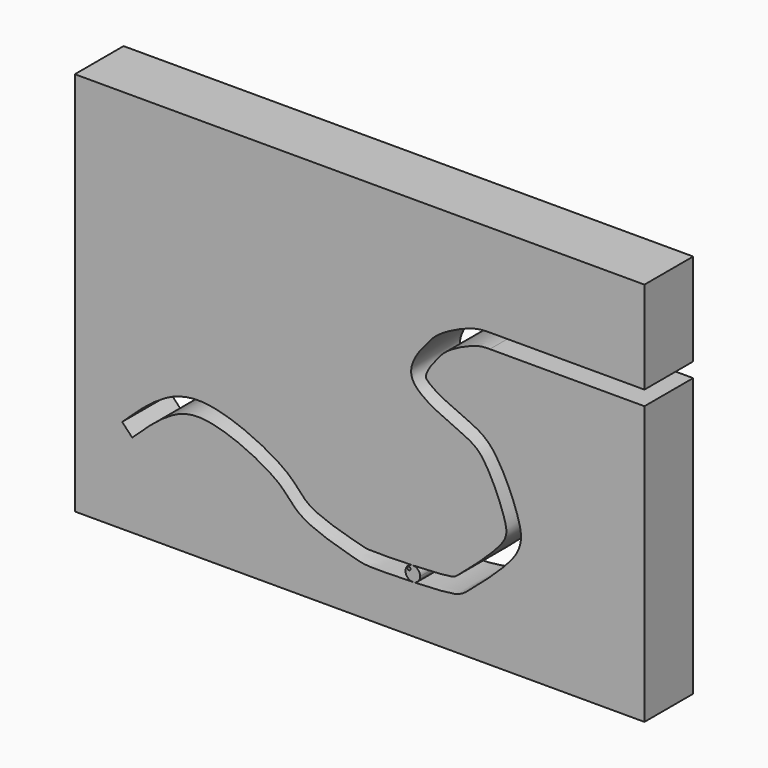
from build123d import *

# Parameters (mm, degrees)
F0_R     = 0.6651863413
F1_DEPTH = 25
F2_DEPTH = 25


# Not quite as in the source:
# - the dataset's text gives a spline's control points without its knots; the knots are read off the source's solid


with BuildPart() as f1:
    # F0 (on Front) → F1 (new body)
    with BuildSketch(Plane.XZ):
        with BuildLine():
            ThreePointArc((122.3084832169, -16.0360134831), (121.3921244993, -13.8776717571), (119.2028572127, -13.0378735352))
            ThreePointArc((119.2028572127, -13.0378735352), (116.3103432648, -16.1416393675), (119.4141089815, -19.0341534395))
            ThreePointArc((119.4141089815, -19.0341534395), (121.4668248597, -18.1196548518), (122.3084832169, -16.0360134831))
        make_face()
        with Locations((117.7324801683, -14.6684795618)):
            Circle(F0_R, mode=Mode.SUBTRACT)
    extrude(amount=F1_DEPTH)


with BuildPart() as f2:
    # F0 (on Front) → F2 (new body)
    with BuildSketch(Plane.XZ):
        with BuildLine():
            Line((4.1454933636, -4.3376127965), (0, 0))
            add(Edge.make_bspline(
                [(0, 0), (4.5037117249, 4.3042355191), (13.7648963192, 13.1552282369), (33.6539795611, 22.3859469816), (70.5260974638, 4.6908661854), (74.9131356895, -6.6840442171), (98.0696827717, -12.5601876128), (100.2690851646, -13.4345128534), (112.4963916518, -13.2741456838), (119.2028572127, -13.0378735352)],
                knots=[0, 0, 0, 0, 0.0640752575, 0.1317608283, 0.2223436266, 0.275722026, 0.3430860694, 0.3769734154, 0.4213979277, 0.4213979277, 0.4213979277, 0.4213979277], degree=3))
            add(Edge.make_bspline(
                [(119.2028572127, -13.0378735352), (125.1175905208, -12.8294945114), (135.8875979213, -12.2260329219), (137.8490544226, -10.5135173732), (157.7784624841, 6.5110943868), (158.2406973488, 14.6134364576), (149.0449665664, 35.7990843084), (140.9804715168, 41.1596578372), (111.9921272876, 52.0827318338), (124.762690675, 68.9964906206), (130.0986463551, 74.7437775542), (143.629972816, 81.2356032201), (148.7753786698, 81.3720077442), (150.9158611298, 81.3720077442)],
                knots=[0.4213979277, 0.4213979277, 0.4213979277, 0.4213979277, 0.4605779012, 0.4949630674, 0.5674303222, 0.6104638131, 0.6784317625, 0.7289830889, 0.802541483, 0.8595384058, 0.9042921665, 0.9601939233, 1, 1, 1, 1], degree=3))
            Line((150.9158611298, 81.3720077442), (214.3666487599, 81.3720077442))
            Line((214.3666487599, 81.3720077442), (214.3666487599, 119.3081084329))
            Line((214.3666487599, 119.3081084329), (-19.4157916641, 119.3081084329))
            Line((-19.4157916641, 119.3081084329), (-19.4157916641, -38.6965889793))
            Line((-19.4157916641, -38.6965889793), (214.3666487599, -38.6965889793))
            Line((214.3666487599, -38.6965889793), (214.3666487599, 75.3720077442))
            Line((214.3666487599, 75.3720077442), (150.9158611298, 75.3720077442))
            add(Edge.make_bspline(
                [(119.4141089799, -19.0341533954), (119.4871101516, -19.0315815327), (120.7551628168, -18.9865960674), (123.2020002243, -18.8892209022), (126.6016258276, -18.721466052), (129.2051336824, -18.5607598165), (131.0997995453, -18.4191431049), (132.4164773871, -18.3058518725), (133.6240077571, -18.1839174375), (134.7173448038, -18.0511427938), (135.7389696275, -17.895900431), (136.7669974316, -17.6868852154), (137.8404453509, -17.3829180115), (138.9380310563, -16.9476296867), (139.9625613283, -16.3985584776), (140.827052172, -15.8155520494), (141.5322803356, -15.2650586357), (142.0407792766, -14.8375029591), (142.438270563, -14.4972905878), (142.8420836155, -14.1508828396), (143.4192170697, -13.6561238308), (144.2024620522, -12.9826805066), (145.0673181917, -12.2355593157), (146.0013266265, -11.4235107422), (147.3241496876, -10.264303774), (149.0949763641, -8.691161638), (152.0635187163, -5.9867519033), (155.0634175663, -3.1175042059), (157.7826477848, -0.2711852119), (159.6172871117, 1.82988094), (160.9426876994, 3.578092876), (161.864848372, 5.0497093246), (162.4790539519, 6.2170852342), (162.9955971863, 7.4607803665), (163.386908628, 8.7726369645), (163.6303999393, 10.1189016964), (163.7228618743, 11.4518844469), (163.6835814445, 12.7316548024), (163.5436641961, 13.9413942325), (163.3329510954, 15.0871340521), (163.1161576384, 16.0068254114), (162.9252065829, 16.7332056778), (162.7195664026, 17.4716247723), (162.4360551739, 18.4166894366), (162.0561419501, 19.5870161779), (161.5002405625, 21.1918771935), (160.7196210908, 23.2706662014), (159.6681934008, 25.8342458833), (158.5248729578, 28.4116494335), (157.3114889212, 30.9458554347), (156.0475232975, 33.3808697793), (154.7457132627, 35.6668674836), (153.4085117355, 37.7623461903), (151.991662503, 39.6641433162), (150.4099177475, 41.3968167785), (148.6511497108, 42.9200771006), (146.7698746062, 44.209111144), (144.8048090764, 45.3123675275), (142.7267705238, 46.3246869099), (140.438462858, 47.3506114125), (137.9747297964, 48.4280612839), (135.4217548209, 49.5672266744), (132.8801749016, 50.7671681076), (130.464059114, 52.0169199809), (128.298049606, 53.2916050203), (126.8152096984, 54.3341822007), (125.8926787851, 55.1057116143), (125.3481084384, 55.6317010892), (124.9614837204, 56.0779002187), (124.7324111989, 56.4110817064), (124.6642598762, 56.5496236369), (124.6469062848, 56.5919977881), (124.6423285594, 56.604558201), (124.6369168484, 56.6223618588), (124.6254672346, 56.6740931465), (124.6168148585, 56.8309541668), (124.6407980996, 57.1110436646), (124.7506534781, 57.6487861525), (125.0802050729, 58.5920803636), (125.8005058034, 59.9854736022), (126.6083870109, 61.2414798545), (127.3291502197, 62.2518120274), (127.8938491077, 63.0028563289), (128.3742714561, 63.6166989958), (128.7582219627, 64.0971795957), (129.0458019743, 64.453161697), (129.3271818406, 64.7988859857), (129.6843642656, 65.2337517538), (130.1035993611, 65.735320869), (130.567326874, 66.2726212921), (131.1425124055, 66.9119050208), (131.7987212915, 67.5854626234), (132.5697497197, 68.2809981123), (133.2950551065, 68.8495639596), (133.9827804314, 69.3348396315), (134.7613012396, 69.8504399686), (135.9102342215, 70.5510874997), (137.4767302693, 71.4187773785), (139.1589871979, 72.2716649361), (140.8857983187, 73.0714834042), (142.302594056, 73.6643488492), (143.3840824883, 74.0773252687), (144.1577631499, 74.3520546179), (144.8839306759, 74.5882634106), (145.540971774, 74.7798881974), (146.1432863223, 74.9327931307), (146.8962108192, 75.095777904), (147.758617804, 75.2335789325), (148.7467949394, 75.3262316993), (149.7679595331, 75.3675621745), (150.5165689591, 75.3720077442), (150.9158611298, 75.3720077442)],
                knots=[0.4213979254, 0.4213979254, 0.4213979254, 0.4213979254, 0.421875, 0.4296875, 0.4375, 0.4453125, 0.44921875, 0.453125, 0.45703125, 0.4609375, 0.46484375, 0.46875, 0.47265625, 0.4765625, 0.48046875, 0.484375, 0.48828125, 0.4921875, 0.494140625, 0.49609375, 0.5, 0.50390625, 0.5078125, 0.51171875, 0.515625, 0.5234375, 0.53125, 0.546875, 0.5546875, 0.5625, 0.5703125, 0.57421875, 0.578125, 0.58203125, 0.5859375, 0.58984375, 0.59375, 0.59765625, 0.6015625, 0.60546875, 0.609375, 0.611328125, 0.61328125, 0.6171875, 0.62109375, 0.625, 0.6328125, 0.640625, 0.6484375, 0.65625, 0.6640625, 0.671875, 0.6796875, 0.6875, 0.6953125, 0.703125, 0.7109375, 0.71875, 0.7265625, 0.734375, 0.7421875, 0.75, 0.7578125, 0.765625, 0.7734375, 0.78125, 0.78515625, 0.7890625, 0.79296875, 0.796875, 0.80078125, 0.8017578125, 0.802734375, 0.8046875, 0.80859375, 0.8125, 0.81640625, 0.8203125, 0.828125, 0.8359375, 0.84375, 0.84765625, 0.8515625, 0.85546875, 0.857421875, 0.859375, 0.861328125, 0.86328125, 0.8671875, 0.87109375, 0.875, 0.8828125, 0.890625, 0.8984375, 0.90234375, 0.90625, 0.9140625, 0.921875, 0.9296875, 0.9375, 0.9453125, 0.94921875, 0.953125, 0.95703125, 0.9609375, 0.96484375, 0.96875, 0.9765625, 0.984375, 0.9921875, 1, 1, 1, 1], degree=3))
            add(Edge.make_bspline(
                [(4.1454933636, -4.3376127965), (5.2437409318, -3.2880082746), (7.4130473658, -1.2150332588), (10.6346217395, 1.7479905226), (13.328983039, 4.0421704542), (15.5108600534, 5.7442358048), (16.8897277858, 6.7471664464), (18.0048744149, 7.5105836164), (19.1135300455, 8.2350503066), (20.4954893224, 9.0654553771), (22.1600034365, 9.9291412323), (24.4128030564, 10.8930416102), (26.7617592156, 11.5664937426), (29.3526802049, 11.9125235338), (31.1092438153, 11.9747900048), (32.6185135441, 11.9179799387), (33.8026291591, 11.8180300331), (35.0658605885, 11.6547378195), (36.8424919842, 11.3539219674), (39.2074188038, 10.826783948), (42.1971171925, 9.9757162304), (45.2681150661, 8.9351274998), (49.3842856633, 7.3371678916), (53.4085483139, 5.4889718545), (57.099619297, 3.5320540573), (59.640004233, 2.0493646835), (61.5133475968, 0.8375436531), (62.8304971794, -0.0906884738), (63.5694491508, -0.6461378338), (64.1054790166, -1.0710734595), (64.4763479102, -1.3766847661), (64.8238613096, -1.6750569086), (65.4841566064, -2.2649459105), (66.359173463, -3.1275277083), (67.4495081459, -4.3249654744), (68.617227829, -5.6566289331), (70.0028678673, -7.1492026464), (71.4329639416, -8.4709854063), (72.7695929433, -9.5133625191), (73.8665488203, -10.2728637672), (75.0695535726, -11.004284465), (76.3089036908, -11.6706590346), (77.586262972, -12.2918209894), (79.3342523936, -13.0700358574), (81.5896831926, -13.9645213472), (84.3430443861, -14.9339157819), (87.061245605, -15.8048884282), (89.6534851435, -16.5766586066), (91.6276841961, -17.1333894197), (93.0427049791, -17.5231249068), (94.0074769688, -17.7862802292), (94.7170841431, -17.9796187266), (95.2200929153, -18.1177136158), (95.5577608478, -18.2113357528), (95.8758779604, -18.3005162078), (96.2867325524, -18.4158262689), (96.7936336212, -18.5562645933), (97.4461681933, -18.7240555173), (98.1680763275, -18.8831391308), (98.945808312, -19.0171782937), (99.7534121549, -19.1172310279), (100.5883223202, -19.186811534), (101.4764122205, -19.2341514561), (102.464072553, -19.2665411051), (103.9552517431, -19.2951732767), (106.1316755542, -19.3064098066), (109.1626871747, -19.2848806165), (112.5021370915, -19.2305099516), (115.9623834061, -19.1470091318), (118.2916543284, -19.0736979571), (119.4141089799, -19.0341533954)],
                knots=[0, 0, 0, 0, 0.015625, 0.03125, 0.046875, 0.0546875, 0.0625, 0.06640625, 0.0703125, 0.078125, 0.0859375, 0.09375, 0.109375, 0.1171875, 0.125, 0.12890625, 0.1328125, 0.13671875, 0.140625, 0.1484375, 0.15625, 0.1640625, 0.171875, 0.1875, 0.1953125, 0.203125, 0.2109375, 0.21484375, 0.21875, 0.220703125, 0.22265625, 0.224609375, 0.2265625, 0.234375, 0.2421875, 0.25, 0.2578125, 0.265625, 0.26953125, 0.2734375, 0.27734375, 0.28125, 0.28515625, 0.2890625, 0.296875, 0.3046875, 0.3125, 0.3203125, 0.328125, 0.33203125, 0.3359375, 0.33984375, 0.341796875, 0.34375, 0.345703125, 0.34765625, 0.3515625, 0.35546875, 0.359375, 0.36328125, 0.3671875, 0.37109375, 0.375, 0.37890625, 0.3828125, 0.390625, 0.3984375, 0.40625, 0.4140625, 0.4213979254, 0.4213979254, 0.4213979254, 0.4213979254], degree=3))
        make_face()
    extrude(amount=F2_DEPTH)


solid = Compound([f1.part, f2.part])
